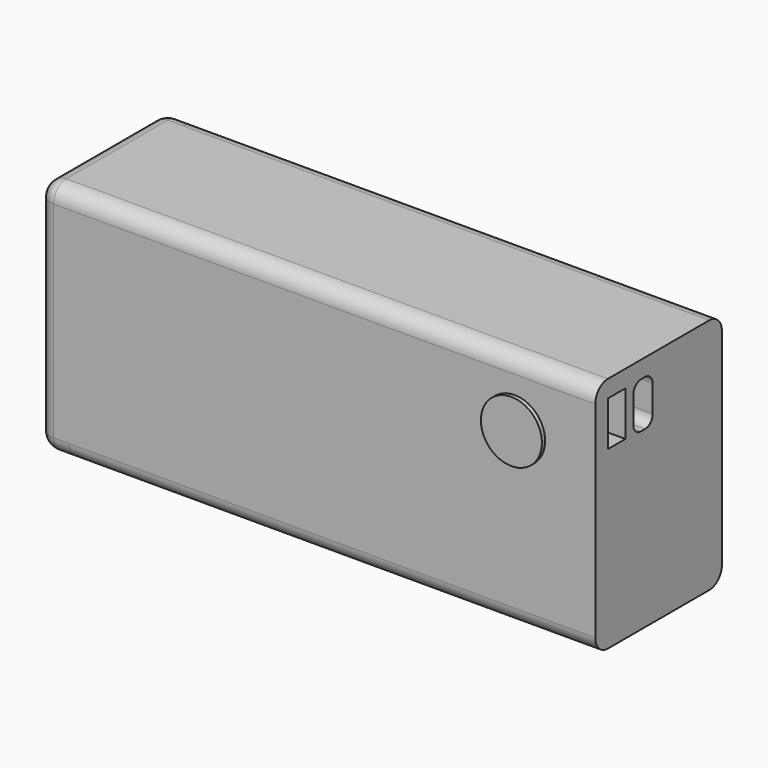
from build123d import *

# Parameters (mm, degrees)
F0_W      = 127
F0_H      = 76.2
F1_DEPTH  = 50.8
F2_R      = 5.08
F3_W      = 7
F3_H      = 14.7
F4_DEPTH  = 16.4
F5_W      = 7
F5_H      = 14.3
F6_DEPTH  = 16.44
F7_W      = 7
F7_H      = 14.3
F8_DEPTH  = 25.4
F9_R      = 9.7907841867
F10_DEPTH = 1.27
F11_DEPTH = 22.352
F13_DEPTH = 25.4
F14_DEPTH = 25.4
F15_DEPTH = 25.4
F16_DEPTH = 10
F17_R     = 5.08


with BuildPart() as f1:
    # F0 (on Front) → F1 (new body)
    with BuildSketch(Plane.XZ):
        Rectangle(F0_W, F0_H)
    extrude(amount=F1_DEPTH)

    # F2
    f2_edges = [f1.edges().sort_by_distance(p)[0] for p in [
        (0, -50.8, 38.1),
        (0, 0, 38.1),
        (0, -50.8, -38.1),
        (0, 0, -38.1),
    ]]
    fillet(f2_edges, radius=F2_R)

    # F3 (on face) → F4 (join)
    with BuildSketch(Plane.YZ.offset(63.5)):
        with BuildLine():
            Line((-5.08, 38.1), (-45.72, 38.1))
            ThreePointArc((-45.72, 38.1), (-49.3121024484, 36.6121024484), (-50.8, 33.02))
            Line((-50.8, 33.02), (-50.8, -33.02))
            ThreePointArc((-50.8, -33.02), (-49.3121024484, -36.6121024484), (-45.72, -38.1))
            Line((-45.72, -38.1), (-5.08, -38.1))
            ThreePointArc((-5.08, -38.1), (-1.4878975516, -36.6121024484), (0, -33.02))
            Line((0, -33.02), (0, 33.02))
            ThreePointArc((0, 33.02), (-1.4878975516, 36.6121024484), (-5.08, 38.1))
        make_face()
        with Locations((-42.22, 25.675587382)):
            Rectangle(F3_W, F3_H, mode=Mode.SUBTRACT)
        with Locations((-42.22, 25.675587382)):
            Rectangle(F3_W, F3_H)
    extrude(amount=-F4_DEPTH)

    # F5 (on face) → F6 (join)
    with BuildSketch(Plane.YZ.offset(63.5)):
        with BuildLine():
            ThreePointArc((-50.8, -33.02), (-49.3121024484, -36.6121024484), (-45.72, -38.1))
            Line((-45.72, -38.1), (-5.08, -38.1))
            ThreePointArc((-5.08, -38.1), (-1.4878975516, -36.6121024484), (0, -33.02))
            Line((0, -33.02), (0, 33.02))
            ThreePointArc((0, 33.02), (-1.4878975516, 36.6121024484), (-5.08, 38.1))
            Line((-5.08, 38.1), (-45.72, 38.1))
            ThreePointArc((-45.72, 38.1), (-49.3121024484, 36.6121024484), (-50.8, 33.02))
            Line((-50.8, 33.02), (-50.8, -33.02))
        make_face()
        with Locations((-42.22, 25.4086919344)):
            Rectangle(F5_W, F5_H, mode=Mode.SUBTRACT)
    extrude(amount=F6_DEPTH)

    # F7 (on face) → F8 (join)
    with BuildSketch(Plane.YZ.offset(79.94)):
        with BuildLine():
            Line((-5.08, 38.1), (-45.72, 38.1))
            ThreePointArc((-45.72, 38.1), (-49.3121024484, 36.6121024484), (-50.8, 33.02))
            Line((-50.8, 33.02), (-50.8, -33.02))
            ThreePointArc((-50.8, -33.02), (-49.3121024484, -36.6121024484), (-45.72, -38.1))
            Line((-45.72, -38.1), (-5.08, -38.1))
            ThreePointArc((-5.08, -38.1), (-1.4878975516, -36.6121024484), (0, -33.02))
            Line((0, -33.02), (0, 33.02))
            ThreePointArc((0, 33.02), (-1.4878975516, 36.6121024484), (-5.08, 38.1))
        make_face()
        with Locations((-42.22, 25.4086919344)):
            Rectangle(F7_W, F7_H, mode=Mode.SUBTRACT)
        with BuildLine():
            Line((-35.5440098792, 20.9126272823), (-35.5440098792, 29.4131070442))
            ThreePointArc((-35.5440098792, 29.4131070442), (-34.6226893957, 31.6373714509), (-32.398424989, 32.5586919344))
            Line((-32.398424989, 32.5586919344), (-30.8212536197, 32.5586919344))
            ThreePointArc((-30.8212536197, 32.5586919344), (-28.6659921506, 31.6659534035), (-27.7732536197, 29.5106919344))
            Line((-27.7732536197, 29.5106919344), (-27.7732536197, 20.9126272823))
            ThreePointArc((-27.7732536197, 20.9126272823), (-28.6659921506, 18.7573658132), (-30.8212536197, 17.8646272823))
            Line((-30.8212536197, 17.8646272823), (-32.4960098792, 17.8646272823))
            ThreePointArc((-32.4960098792, 17.8646272823), (-34.6512713483, 18.7573658132), (-35.5440098792, 20.9126272823))
        make_face(mode=Mode.SUBTRACT)
    extrude(amount=F8_DEPTH)

    # F9 (on face) → F10 (join)
    with BuildSketch(Plane.XZ.offset(50.8)):
        with Locations((79.4515386224, 17.386501655)):
            Circle(F9_R)
    extrude(amount=F10_DEPTH)

    # F11 (add): a face of the model
    f11_faces = [f1.faces().sort_by_distance(p)[0] for p in [
        (79.4515386224, -52.07, 17.386501655),
    ]]
    extrude(f11_faces, amount=-F11_DEPTH)

    # F12 (on face) → F13 (join)
    with BuildSketch(Plane(origin=(-63.5, 0, 0), x_dir=(0, -1, 0), z_dir=(-1, 0, 0))):
        with BuildLine():
            Line((20.797392028, 16.5488310158), (19.2076092115, 16.5488310158))
            ThreePointArc((19.2076092115, 16.5488310158), (16.5135323752, 15.4329078521), (15.3976092115, 12.7388310158))
            Line((15.3976092115, 12.7388310158), (15.3976092115, 11.0805211589))
            Line((15.3976092115, 11.0805211589), (15.6854148954, 11.0805211589))
            Line((15.6854148954, 11.0805211589), (24.607392028, 11.0805211589))
            Line((24.607392028, 11.0805211589), (24.607392028, 12.7388310158))
            ThreePointArc((24.607392028, 12.7388310158), (23.4914688643, 15.4329078521), (20.797392028, 16.5488310158))
        make_face()
    extrude(amount=-F13_DEPTH)

    # F12 (on face) → F14 (join)
    with BuildSketch(Plane(origin=(-63.5, 0, 0), x_dir=(0, -1, 0), z_dir=(-1, 0, 0))):
        with BuildLine():
            Line((20.797392028, 16.5488310158), (19.2076092115, 16.5488310158))
            ThreePointArc((19.2076092115, 16.5488310158), (16.5135323752, 15.4329078521), (15.3976092115, 12.7388310158))
            Line((15.3976092115, 12.7388310158), (15.3976092115, 11.0805211589))
            Line((15.3976092115, 11.0805211589), (15.6854148954, 11.0805211589))
            Line((15.6854148954, 11.0805211589), (24.607392028, 11.0805211589))
            Line((24.607392028, 11.0805211589), (24.607392028, 12.7388310158))
            ThreePointArc((24.607392028, 12.7388310158), (23.4914688643, 15.4329078521), (20.797392028, 16.5488310158))
        make_face()
    extrude(amount=-F14_DEPTH)

    # F12 (on face) → F15 (join)
    with BuildSketch(Plane(origin=(-63.5, 0, 0), x_dir=(0, -1, 0), z_dir=(-1, 0, 0))):
        with BuildLine():
            Line((20.797392028, 16.5488310158), (19.2076092115, 16.5488310158))
            ThreePointArc((19.2076092115, 16.5488310158), (16.5135323752, 15.4329078521), (15.3976092115, 12.7388310158))
            Line((15.3976092115, 12.7388310158), (15.3976092115, 11.0805211589))
            Line((15.3976092115, 11.0805211589), (15.6854148954, 11.0805211589))
            Line((15.6854148954, 11.0805211589), (24.607392028, 11.0805211589))
            Line((24.607392028, 11.0805211589), (24.607392028, 12.7388310158))
            ThreePointArc((24.607392028, 12.7388310158), (23.4914688643, 15.4329078521), (20.797392028, 16.5488310158))
        make_face()
    extrude(amount=-F15_DEPTH)

    # F12 (on face) → F16 (join)
    with BuildSketch(Plane(origin=(-63.5, 0, 0), x_dir=(0, -1, 0), z_dir=(-1, 0, 0))):
        with BuildLine():
            ThreePointArc((50.8, 33.02), (49.3121024484, 36.6121024484), (45.72, 38.1))
            Line((45.72, 38.1), (5.08, 38.1))
            ThreePointArc((5.08, 38.1), (1.4878975516, 36.6121024484), (0, 33.02))
            Line((0, 33.02), (0, -33.02))
            ThreePointArc((0, -33.02), (1.4878975516, -36.6121024484), (5.08, -38.1))
            Line((5.08, -38.1), (45.72, -38.1))
            ThreePointArc((45.72, -38.1), (49.3121024484, -36.6121024484), (50.8, -33.02))
            Line((50.8, -33.02), (50.8, 33.02))
        make_face()
        with BuildLine():
            ThreePointArc((15.3976092115, 12.7388310158), (16.5135323752, 15.4329078521), (19.2076092115, 16.5488310158))
            Line((19.2076092115, 16.5488310158), (20.797392028, 16.5488310158))
            ThreePointArc((20.797392028, 16.5488310158), (23.4914688643, 15.4329078521), (24.607392028, 12.7388310158))
            Line((24.607392028, 12.7388310158), (24.607392028, 11.0805211589))
            Line((24.607392028, 11.0805211589), (15.6854148954, 11.0805211589))
            Line((15.6854148954, 11.0805211589), (15.3976092115, 11.0805211589))
            Line((15.3976092115, 11.0805211589), (15.3976092115, 12.7388310158))
        make_face(mode=Mode.SUBTRACT)
    extrude(amount=F16_DEPTH)

    # F17
    f17_edges = [f1.edges().sort_by_distance(p)[0] for p in [
        (-73.5, -25.4, 38.1),
        (-73.5, 0, 0),
        (-73.5, -25.4, -38.1),
        (-73.5, -50.8, 0),
        (-73.5, -49.312102, 36.612102),
        (-73.5, -1.487898, 36.612102),
        (-73.5, -49.312102, -36.612102),
        (-73.5, -1.487898, -36.612102),
    ]]
    fillet(f17_edges, radius=F17_R)


solid = f1.part
